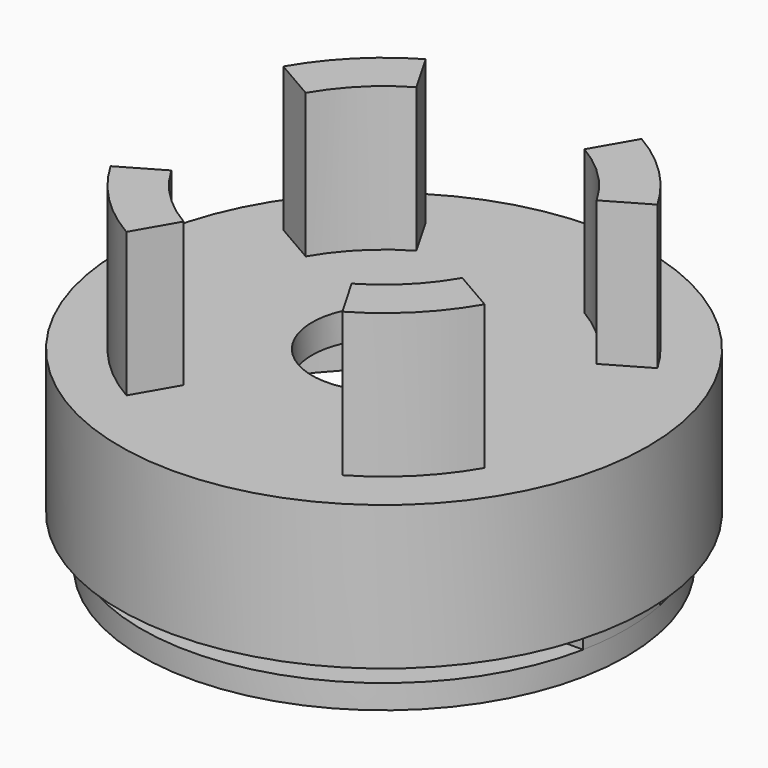
from build123d import *

# Parameters (mm, degrees)
F0_R      = 27.5
F1_DEPTH  = 15
F2_R      = 25.25
F3_DEPTH  = 12
F4_R      = 25.25
F4_R_2    = 21.25
F5_DEPTH  = 2
F6_R      = 7.5
F7_DEPTH  = 3
F8_R      = 22.5
F8_R_2    = 17.5
F9_DEPTH  = 15
F11_DEPTH = 15
F13_DEPTH = 2.5
F14_R     = 1.75
F15_DEPTH = 10
F16_R     = 25.25
F17_DEPTH = 2.5


# Not quite as in the source:
# - after a boolean that leaves OpenCascade's solid faulty, fix() repairs it


with BuildPart() as f1:
    # F0 (on Top) → F1 (new body)
    with BuildSketch(Plane.XY):
        Circle(F0_R)
    extrude(amount=F1_DEPTH)

    # F2 (on face) → F3 (cut)
    with BuildSketch(Plane(origin=(0, 0, 0), x_dir=(1, 0, 0), z_dir=(0, 0, -1))):
        Circle(F2_R)
    extrude(amount=-F3_DEPTH, mode=Mode.SUBTRACT)

    # F4 (on face) → F5 (join)
    with BuildSketch(Plane(origin=(0, 0, 12), x_dir=(1, 0, 0), z_dir=(0, 0, -1))):
        Circle(F4_R)
        Circle(F4_R_2, mode=Mode.SUBTRACT)
    extrude(amount=F5_DEPTH)

    # F6 (on face) → F7 (cut, through all)
    with BuildSketch(Plane.XY.offset(15)):
        Circle(F6_R)
    extrude(amount=-F7_DEPTH, mode=Mode.SUBTRACT)

    # F8 (on face) → F9 (join)
    with BuildSketch(Plane.XY.offset(15)):
        Circle(F8_R)
        Circle(F8_R_2, mode=Mode.SUBTRACT)
    extrude(amount=F9_DEPTH)

    # F10 (on face) → F11 (cut, through all)
    with BuildSketch(Plane.XY.offset(30)):
        with BuildLine():
            ThreePointArc((-15.1554445662, -8.75), (-17.5, 0), (-15.1554445662, 8.75))
            Line((-15.1554445662, 8.75), (-19.4855715851, 11.25))
            ThreePointArc((-19.4855715851, 11.25), (-22.5, 0), (-19.4855715851, -11.25))
            Line((-19.4855715851, -11.25), (-15.1554445662, -8.75))
        make_face()
        with BuildLine():
            ThreePointArc((8.75, -15.1554445662), (0, -17.5), (-8.75, -15.1554445662))
            Line((-8.75, -15.1554445662), (-11.25, -19.4855715851))
            ThreePointArc((-11.25, -19.4855715851), (0, -22.5), (11.25, -19.4855715851))
            Line((11.25, -19.4855715851), (8.75, -15.1554445662))
        make_face()
        with BuildLine():
            Line((19.4855715851, 11.25), (15.1554445662, 8.75))
            ThreePointArc((15.1554445662, 8.75), (16.9037019601, 4.5293332893), (17.5, 0))
            ThreePointArc((17.5, 0), (16.9037019601, -4.5293332893), (15.1554445662, -8.75))
            Line((15.1554445662, -8.75), (19.4855715851, -11.25))
            ThreePointArc((19.4855715851, -11.25), (21.7333310915, -5.8234285148), (22.5, 0))
            ThreePointArc((22.5, 0), (21.7333310915, 5.8234285148), (19.4855715851, 11.25))
        make_face()
        with BuildLine():
            ThreePointArc((-8.75, 15.1554445662), (0, 17.5), (8.75, 15.1554445662))
            Line((8.75, 15.1554445662), (11.25, 19.4855715851))
            ThreePointArc((11.25, 19.4855715851), (0, 22.5), (-11.25, 19.4855715851))
            Line((-11.25, 19.4855715851), (-8.75, 15.1554445662))
        make_face()
    extrude(amount=-F11_DEPTH, mode=Mode.SUBTRACT)



with BuildPart() as f13:
    # F12 (on Top) → F13 (new body)
    with BuildSketch(Plane.XY):
        with BuildLine():
            Line((-24.75, -5), (-8.6602540378, -5))
            ThreePointArc((-8.6602540378, -5), (0, -10), (8.6602540378, -5))
            Line((8.6602540378, -5), (24.75, -5))
            ThreePointArc((24.75, -5), (25.25, 0), (24.75, 5))
            Line((24.75, 5), (8.6602540378, 5))
            ThreePointArc((8.6602540378, 5), (0, 10), (-8.6602540378, 5))
            Line((-8.6602540378, 5), (-24.75, 5))
            ThreePointArc((-24.75, 5), (-25.25, 0), (-24.75, -5))
        make_face()
    extrude(amount=-F13_DEPTH)


with BuildPart() as f1_1:
    add(f1.part)

    add(f13.part)  # F15 merges F13
    # F14 (on face) → F15 (join)
    with BuildSketch(Plane.XY):
        with Locations((-19.5, 0)):
            Circle(F14_R)
        with Locations((19.5, 0)):
            Circle(F14_R)
    extrude(amount=F15_DEPTH)

    # F16 (on face) → F17 (join)
    with BuildSketch(Plane(origin=(0, 0, -2.5), x_dir=(1, 0, 0), z_dir=(0, 0, -1))):
        Circle(F16_R)
    extrude(amount=F17_DEPTH)

    add(f1_1.part.fix(), mode=Mode.REPLACE)


solid = f1_1.part
